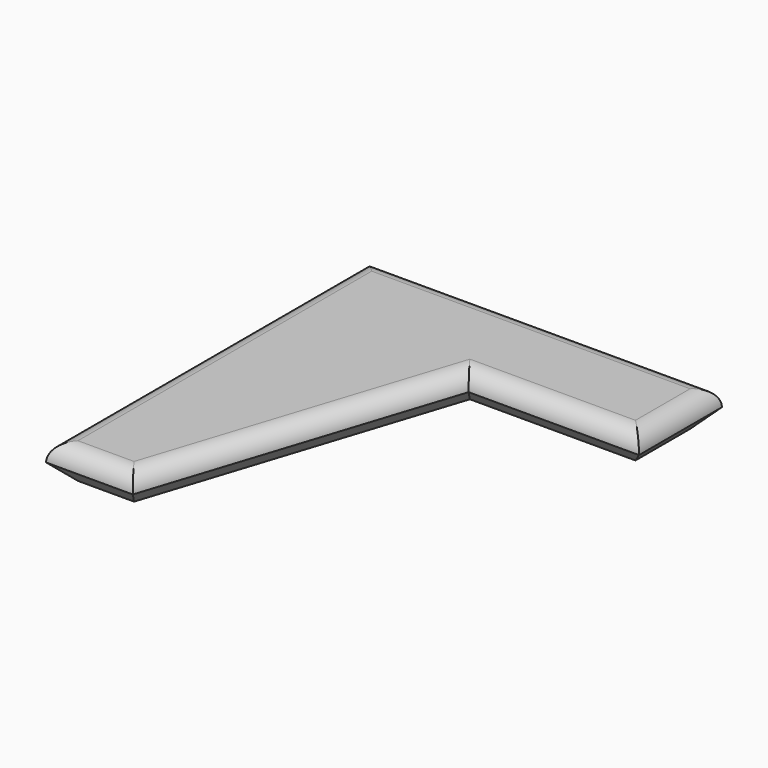
from build123d import *

# Parameters (mm, degrees)
F1_DEPTH = 10
F2_R     = 5
F3_SIZE  = 4.99999


# Not quite as in the source:
# - a fillet or chamfer is up to 0.001 mm smaller than in the source, because OpenCascade refuses the exact size


with BuildPart() as f1:
    # F0 (on Top) → F1 (new body)
    with BuildSketch(Plane.XY):
        Polygon((42.2499991953, 60.7764059144), (-57.7500008047, 60.7764059144), (-57.7500008047, -53.026408835), (-33.2429584743, -53.026408835), (-5.9190154745, 31.4806343348), (42.2499991953, 31.4806343348), align=None)
    extrude(amount=F1_DEPTH)

    # F2
    f2_edges = [f1.edges().sort_by_distance(p)[0] for p in [
        (-57.750001, 3.874999, 10),
        (-19.580987, -10.772887, 10),
        (-45.49648, -53.026409, 10),
        (18.165492, 31.480634, 10),
        (-7.750001, 60.776406, 10),
        (42.249999, 46.12852, 10),
    ]]
    fillet(f2_edges, radius=F2_R)

    # F3 (size 5 in the source; OpenCascade refuses exactly that, so slightly less here)
    f3_edges = [f1.edges().sort_by_distance(p)[0] for p in [
        (18.165492, 31.480634, 0),
        (42.249999, 46.12852, 0),
        (-7.750001, 60.776406, 0),
        (-57.750001, 3.874999, 0),
        (-45.49648, -53.026409, 0),
        (-19.580987, -10.772887, 0),
    ]]
    chamfer(f3_edges, length=F3_SIZE)


solid = f1.part
